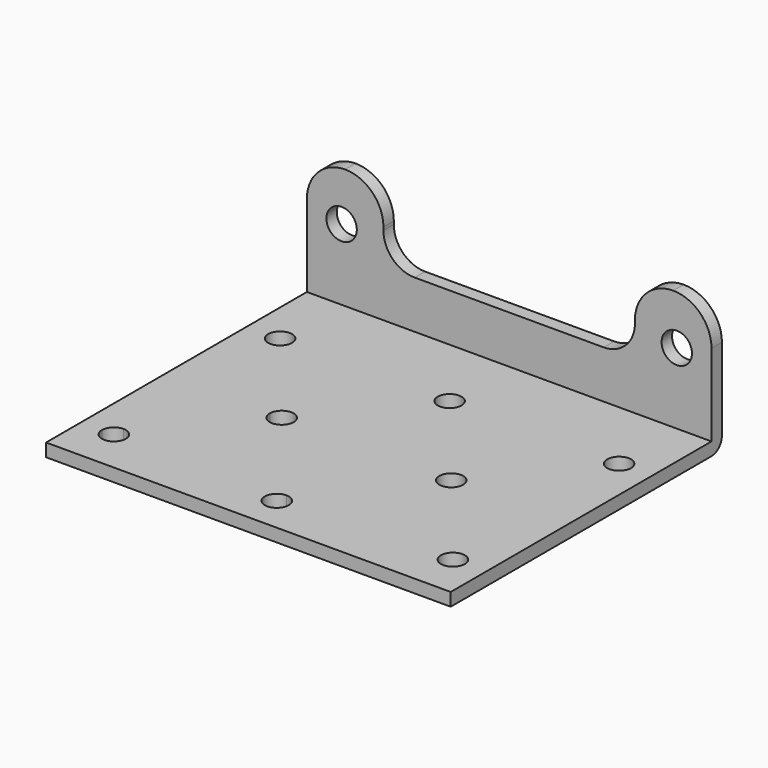
from build123d import *

# Parameters (mm, degrees)
F0_R     = 4.365625
F0_W     = 148
F0_H     = 4.7625
F1_DEPTH = 4.7625
F2_DEPTH = 44
F3_R     = 4.7625
F4_R     = 5.55625
F5_DEPTH = 6.35


# Not quite as in the source:
# - a feature names something its author has since deleted; it is built from what else it names


with BuildPart() as f1:
    # F0 (on Top) → F1 (new body)
    with BuildSketch(Plane.XY):
        with BuildLine():
            Line((-31, -12.365625), (-31, -62))
            Line((-31, -62), (0, -62))
            Line((0, -62), (74, -62))
            Line((74, -62), (74, 57.2375))
            Line((74, 57.2375), (-74, 57.2375))
            Line((-74, 57.2375), (-74, -8))
            Line((-74, -8), (-62, -8))
            Line((-62, -8), (-35.365625, -8))
            ThreePointArc((-35.365625, -8), (-31, -3.634375), (-26.634375, -8))
            ThreePointArc((-26.634375, -8), (-27.9130369584, -11.0869630416), (-31, -12.365625))
        make_face()
        with BuildLine():
            ThreePointArc((4.365625, -49), (3.0869630416, -52.0869630416), (0, -53.365625))
            ThreePointArc((0, -53.365625), (-4.365625, -49), (0, -44.634375))
            ThreePointArc((0, -44.634375), (3.0869630416, -45.9130369584), (4.365625, -49))
        make_face(mode=Mode.SUBTRACT)
        with Locations((62, -46)):
            Circle(F0_R, mode=Mode.SUBTRACT)
        with Locations((31, -8)):
            Circle(F0_R, mode=Mode.SUBTRACT)
        with BuildLine():
            ThreePointArc((-57.634375, 30), (-58.9130369584, 26.9130369584), (-62, 25.634375))
            ThreePointArc((-62, 25.634375), (-65.0869630416, 33.0869630416), (-57.634375, 30))
        make_face(mode=Mode.SUBTRACT)
        with BuildLine():
            ThreePointArc((4.365625, 30), (3.0869630416, 26.9130369584), (0, 25.634375))
            ThreePointArc((0, 25.634375), (-3.0869630416, 33.0869630416), (4.365625, 30))
        make_face(mode=Mode.SUBTRACT)
        with Locations((62, 30)):
            Circle(F0_R, mode=Mode.SUBTRACT)
        with Locations((0, 59.61875)):
            Rectangle(F0_W, F0_H)
        with BuildLine():
            Line((-62, -50.365625), (-62, -62))
            Line((-62, -62), (-31, -62))
            Line((-31, -62), (-31, -12.365625))
            ThreePointArc((-31, -12.365625), (-34.0869630416, -11.0869630416), (-35.365625, -8))
            Line((-35.365625, -8), (-62, -8))
            Line((-62, -8), (-62, -41.634375))
            ThreePointArc((-62, -41.634375), (-58.9130369584, -42.9130369584), (-57.634375, -46))
            ThreePointArc((-57.634375, -46), (-58.9130369584, -49.0869630416), (-62, -50.365625))
        make_face()
        with BuildLine():
            Line((-74, -8), (-74, -46))
            Line((-74, -46), (-66.365625, -46))
            ThreePointArc((-66.365625, -46), (-65.0869630416, -42.9130369584), (-62, -41.634375))
            Line((-62, -41.634375), (-62, -8))
            Line((-62, -8), (-74, -8))
        make_face()
        with BuildLine():
            Line((-74, -46), (-74, -62))
            Line((-74, -62), (-62, -62))
            Line((-62, -62), (-62, -50.365625))
            ThreePointArc((-62, -50.365625), (-65.0869630416, -49.0869630416), (-66.365625, -46))
            Line((-66.365625, -46), (-74, -46))
        make_face()
    extrude(amount=-F1_DEPTH)

    # F0 (on Top) → F2 (join)
    with BuildSketch(Plane.XY):
        with Locations((0, 59.61875)):
            Rectangle(F0_W, F0_H)
    extrude(amount=F2_DEPTH)

    # F3
    f3_edges = [f1.edges().sort_by_distance(p)[0] for p in [
        (0, 62, -4.7625),
    ]]
    fillet(f3_edges, radius=F3_R)

    # F4 (on face) → F5 (cut)
    with BuildSketch(Plane(origin=(0, 62, 0), x_dir=(-1, 0, 0), z_dir=(0, 1, 0))):
        with BuildLine():
            ThreePointArc((-60, 44), (-50.1005050634, 39.8994949366), (-46, 30))
            Line((-46, 30), (-46, 28.8925))
            ThreePointArc((-46, 28.8925), (-42.652230509, 20.810269491), (-34.57, 17.4625))
            Line((-34.57, 17.4625), (0, 17.4625))
            Line((0, 17.4625), (34.57, 17.4625))
            ThreePointArc((34.57, 17.4625), (42.652230509, 20.810269491), (46, 28.8925))
            Line((46, 28.8925), (46, 30))
            ThreePointArc((46, 30), (50.1005050634, 39.8994949366), (60, 44))
            Line((60, 44), (59.7125, 44))
            Line((59.7125, 44), (-60, 44))
        make_face()
        with BuildLine():
            Line((74, 44), (60, 44))
            ThreePointArc((60, 44), (69.8994949366, 39.8994949366), (74, 30))
            Line((74, 30), (74, 44))
        make_face()
        with Locations((-61.3, 26)):
            Circle(F4_R)
        with Locations((61.3, 26)):
            Circle(F4_R)
        with BuildLine():
            ThreePointArc((-74, 30), (-69.8994949366, 39.8994949366), (-60, 44))
            Line((-60, 44), (-74, 44))
            Line((-74, 44), (-74, 30))
        make_face()
    extrude(amount=-F5_DEPTH, mode=Mode.SUBTRACT)


solid = f1.part
